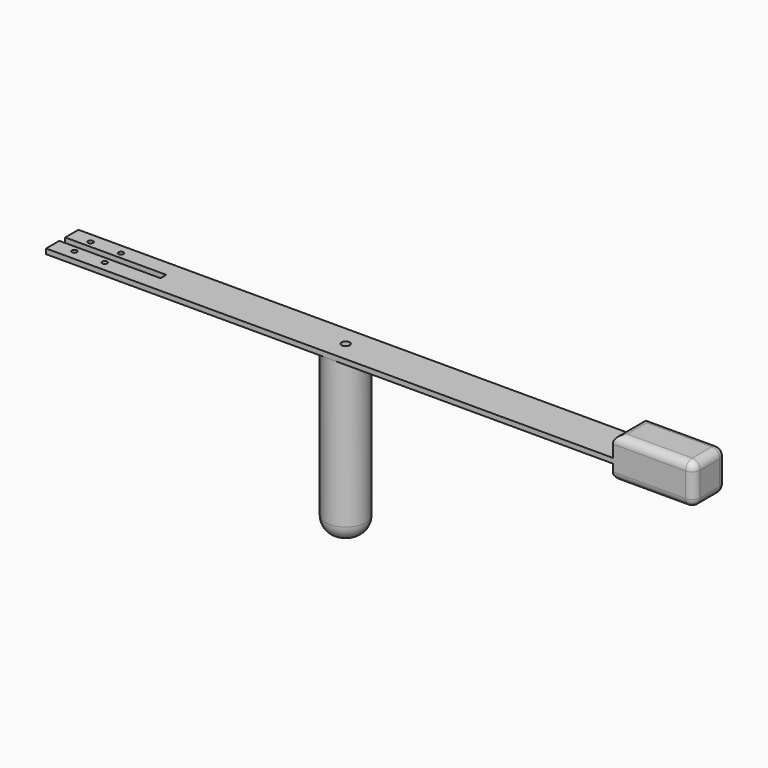
from build123d import *

# Parameters (mm, degrees)
F0_W          = 203.2
F0_H          = 3.175
F1_DEPTH      = 25.4
F2_R          = 1.5875
F3_DEPTH      = 25.4
F4_R          = 12.7
F5_DEPTH      = 101.6
F6_R          = 10.16
F7_R          = 2.54
F8_DEPTH      = 254
F9_W          = 63.5
F9_H          = 4.572
F10_DEPTH     = 25.4
F11_W         = 203.2
F11_H         = 25.4
F12_DEPTH     = 3.175
F13_W         = 50.8
F13_H         = 25.4
F14_DEPTH     = 12.7
F15_DEPTH     = 12.7
F16_R         = 5.08
F17_T1_DEPTH  = 15.24
F17_S5_W      = 5.08
F17_S5_H      = 5.08
F17_T6_DEPTH  = 5.08
F17_S11_W     = 5.08
F17_S11_H     = 5.08
F17_T12_DEPTH = 5.08
F17_S17_W     = 5.08
F17_S17_H     = 5.08
F17_T18_DEPTH = 5.08
F17_S23_W     = 5.08
F17_S23_H     = 5.08
F17_T24_DEPTH = 5.08


# Not quite as in the source:
# - a fillet or chamfer that OpenCascade refuses, or shapes differently, is made with other operations: its cross-section is extruded or revolved along the edge and cut away or added


with BuildPart() as f1:
    # F0 (on Front) → F1 (new body)
    with BuildSketch(Plane.XZ):
        with Locations((101.6, 1.5875)):
            Rectangle(F0_W, F0_H)
    extrude(amount=F1_DEPTH)

    # F2 (on face) → F3 (cut)
    with BuildSketch(Plane.XY.offset(3.175)):
        with Locations((12.7, -19.05)):
            Circle(F2_R)
        with Locations((12.7, -6.35)):
            Circle(F2_R)
        with Locations((31.75, -6.35)):
            Circle(F2_R)
        with Locations((31.75, -19.05)):
            Circle(F2_R)
    extrude(amount=-F3_DEPTH, mode=Mode.SUBTRACT)

    # F4 (on face) → F5 (join)
    with BuildSketch(Plane(origin=(0, 0, 0), x_dir=(1, 0, 0), z_dir=(0, 0, -1))):
        with Locations((177.8, 12.7)):
            Circle(F4_R)
    extrude(amount=F5_DEPTH)

    # F6
    f6_edges = [f1.edges().sort_by_distance(p)[0] for p in [
        (165.1, -12.7, -101.6),
    ]]
    fillet(f6_edges, radius=F6_R)

    # F7 (on face) → F8 (cut)
    with BuildSketch(Plane(origin=(0, 0, -101.6), x_dir=(1, 0, 0), z_dir=(0, 0, -1))):
        with Locations((177.8, 12.7)):
            Circle(F7_R)
    extrude(amount=-F8_DEPTH, mode=Mode.SUBTRACT)

    # F9 (on face) → F10 (cut)
    with BuildSketch(Plane.XY.offset(3.175)):
        with Locations((31.75, -12.7)):
            Rectangle(F9_W, F9_H)
    extrude(amount=-F10_DEPTH, mode=Mode.SUBTRACT)

    # F11 (on face) → F12 (join)
    with BuildSketch(Plane.XY.offset(3.175)):
        with Locations((304.8, -12.7)):
            Rectangle(F11_W, F11_H)
    extrude(amount=-F12_DEPTH)

    # F13 (on face) → F14 (join)
    with BuildSketch(Plane.XY.offset(3.175)):
        with Locations((381, -12.7)):
            Rectangle(F13_W, F13_H)
    extrude(amount=F14_DEPTH)

    # F13 (on face) → F15 (join)
    with BuildSketch(Plane.XY.offset(3.175)):
        with Locations((381, -12.7)):
            Rectangle(F13_W, F13_H)
    extrude(amount=-F15_DEPTH)

    # F16
    f16_edges = [f1.edges().sort_by_distance(p)[0] for p in [
        (406.4, -12.7, 15.875),
        (406.4, -12.7, -9.525),
        (355.6, -12.7, 15.875),
        (355.6, -12.7, -9.525),
        (381, -25.4, 15.875),
        (381, -25.4, -9.525),
        (381, 0, 15.875),
        (381, 0, -9.525),
    ]]
    fillet(f16_edges, radius=F16_R)

    # F17: fillet of radius 5.08 on 2 edges, made by hand

    # F17_s2 → F17_t1 (cut)
    with BuildSketch(Plane.XY.offset(-4.445)):
        with BuildLine():
            ThreePointArc((401.32, 0), (404.9121024484, -1.4878975516), (406.4, -5.08))
            Line((406.4, -5.08), (406.4, 0))
            Line((406.4, 0), (401.32, 0))
        make_face()
        with BuildLine():
            ThreePointArc((401.32, -25.4), (404.9121024484, -23.9121024484), (406.4, -20.32))
            Line((406.4, -20.32), (406.4, -25.4))
            Line((406.4, -25.4), (401.32, -25.4))
        make_face()
    extrude(amount=F17_T1_DEPTH, mode=Mode.SUBTRACT)


with BuildPart() as f17_tool4:
    # F17_s5 → F17_t6 (new body)
    with BuildSketch(Plane.XZ.offset(20.32)):
        with Locations((403.86, 13.335)):
            Rectangle(F17_S5_W, F17_S5_H)
    extrude(amount=F17_T6_DEPTH)

    # F17_s7 → F17_t8 (revolve, cut)
    with BuildSketch(Plane(origin=(401.32, -20.32, 10.795), x_dir=(-0.7071067812, 0, -0.7071067812), z_dir=(-0.7071067812, 0, 0.7071067812))):
        with BuildLine():
            ThreePointArc((0, -5.08), (5.08, 0), (0, 5.08))
            Line((0, 5.08), (0, -5.08))
        make_face()
    revolve(axis=Axis((401.32, -20.32, 10.795), (0, -1, 0)), mode=Mode.SUBTRACT)


with BuildPart() as f1_1:
    add(f1.part)

    # F17_t3: cut F17_tool4
    add(f17_tool4.part, mode=Mode.SUBTRACT)


with BuildPart() as f17_tool10:
    # F17_s11 → F17_t12 (new body)
    with BuildSketch(Plane.XZ.offset(5.08)):
        with Locations((403.86, 13.335)):
            Rectangle(F17_S11_W, F17_S11_H)
    extrude(amount=-F17_T12_DEPTH)

    # F17_s13 → F17_t14 (revolve, cut)
    with BuildSketch(Plane(origin=(401.32, -5.08, 10.795), x_dir=(-0.7071067812, 0, -0.7071067812), z_dir=(0.7071067812, 0, -0.7071067812))):
        with BuildLine():
            ThreePointArc((0, -5.08), (5.08, 0), (0, 5.08))
            Line((0, 5.08), (0, -5.08))
        make_face()
    revolve(axis=Axis((401.32, -5.08, 10.795), (0, 1, 0)), mode=Mode.SUBTRACT)


with BuildPart() as f1_2:
    add(f1_1.part)

    # F17_t9: cut F17_tool10
    add(f17_tool10.part, mode=Mode.SUBTRACT)


with BuildPart() as f17_tool16:
    # F17_s17 → F17_t18 (new body)
    with BuildSketch(Plane.XZ.offset(5.08)):
        with Locations((403.86, -6.985)):
            Rectangle(F17_S17_W, F17_S17_H)
    extrude(amount=-F17_T18_DEPTH)

    # F17_s19 → F17_t20 (revolve, cut)
    with BuildSketch(Plane(origin=(401.32, -5.08, -4.445), x_dir=(-0.7071067812, 0, 0.7071067812), z_dir=(-0.7071067812, 0, -0.7071067812))):
        with BuildLine():
            ThreePointArc((0, -5.08), (5.08, 0), (0, 5.08))
            Line((0, 5.08), (0, -5.08))
        make_face()
    revolve(axis=Axis((401.32, -5.08, -4.445), (0, 1, 0)), mode=Mode.SUBTRACT)


with BuildPart() as f1_3:
    add(f1_2.part)

    # F17_t15: cut F17_tool16
    add(f17_tool16.part, mode=Mode.SUBTRACT)


with BuildPart() as f17_tool22:
    # F17_s23 → F17_t24 (new body)
    with BuildSketch(Plane.XZ.offset(20.32)):
        with Locations((403.86, -6.985)):
            Rectangle(F17_S23_W, F17_S23_H)
    extrude(amount=F17_T24_DEPTH)

    # F17_s25 → F17_t26 (revolve, cut)
    with BuildSketch(Plane(origin=(401.32, -20.32, -4.445), x_dir=(-0.7071067812, 0, 0.7071067812), z_dir=(0.7071067812, 0, 0.7071067812))):
        with BuildLine():
            ThreePointArc((0, -5.08), (5.08, 0), (0, 5.08))
            Line((0, 5.08), (0, -5.08))
        make_face()
    revolve(axis=Axis((401.32, -20.32, -4.445), (0, -1, 0)), mode=Mode.SUBTRACT)


with BuildPart() as f1_4:
    add(f1_3.part)

    # F17_t21: cut F17_tool22
    add(f17_tool22.part, mode=Mode.SUBTRACT)


solid = f1_4.part
